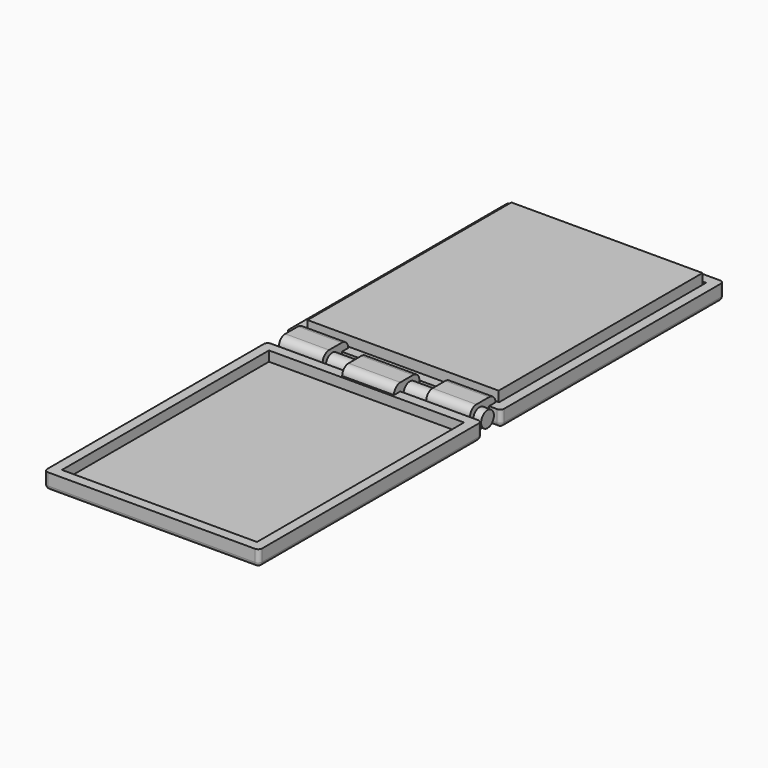
from build123d import *

# Parameters (mm, degrees)
F0_W      = 24
F0_H      = 32
F1_DEPTH  = 2.1
F3_W      = 27.0000016689
F3_H      = 35.0000016689
F3_W_2    = 24
F3_H_2    = 32
F4_DEPTH  = 4
F6_OFFSET = 0.25
F7_R      = 0.5
F5_W      = 35.0000016689
F5_H      = 2
F8_DEPTH  = 27.0000016689
F11_W     = 6.5
F11_H     = 2.9999983311
F11_H_2   = 1
F12_DEPTH = 3
F11_W_2   = 5.5000003338
F11_W_3   = 5.5000004172
F13_R     = 1
F14_DEPTH = 25
F15_R     = 1
F15_2_R   = 1
F15_3_R   = 1


with BuildPart() as f1:
    # F0 (on Top) → F1 (new body)
    with BuildSketch(Plane.XY):
        with Locations((12, 16)):
            Rectangle(F0_W, F0_H)
    extrude(amount=F1_DEPTH)


with BuildPart() as f4:
    # F3 (on offset) → F4 (new body)
    with BuildSketch(Plane.XY.offset(-1)):
        with Locations((12, 16)):
            Rectangle(F3_W, F3_H)
        with Locations((12, 16)):
            Rectangle(F3_W_2, F3_H_2, mode=Mode.SUBTRACT)
        with Locations((12, 16)):
            Rectangle(F3_W_2, F3_H_2)
    extrude(amount=F4_DEPTH)

    # F6: cut F1, made larger all round first
    f6_tool = offset(f1.part, amount=F6_OFFSET, kind=Kind.INTERSECTION, mode=Mode.PRIVATE)
    add(f6_tool, mode=Mode.SUBTRACT)

    # F7
    f7_edges = [f4.edges().sort_by_distance(p)[0] for p in [
        (-1.500001, -1.500001, 1),
        (25.500001, -1.500001, 1),
        (25.500001, 33.500001, 1),
        (-1.500001, 33.500001, 1),
        (-1.500001, 16, 3),
        (12, 33.500001, 3),
        (12, 33.500001, -1),
        (-1.500001, 16, -1),
        (25.500001, 16, 3),
        (25.500001, 16, -1),
        (12, -1.500001, 3),
        (12, -1.500001, -1),
    ]]
    fillet(f7_edges, radius=F7_R)

    # F5 (on face) → F8 (cut, through all)
    with BuildSketch(Plane.YZ.offset(25.5000008345)):
        with Locations((16, 2)):
            Rectangle(F5_W, F5_H)
    extrude(amount=-F8_DEPTH, mode=Mode.SUBTRACT)


with BuildPart() as f10_1:
    # F10: instance of F4
    add(f4.part.mirror(Plane.XZ.offset(3)))


with BuildPart() as f12:
    # F11 (on offset) → F12 (new body)
    with BuildSketch(Plane.XY.offset(-1)):
        with Locations((11.9999995828, -3)):
            Rectangle(F11_W, F11_H)
        with Locations((11.9999995828, -4.9999991655)):
            Rectangle(F11_W, F11_H_2)
    extrude(amount=F12_DEPTH)

    # F15
    f15_edges = [f12.edges().sort_by_distance(p)[0] for p in [
        (12, -5.499999, 2),
        (12, -1.500001, 2),
    ]]
    fillet(f15_edges, radius=F15_R)


with BuildPart() as f12b:
    # F11 (on offset) → F12, piece 2 (new body)
    with BuildSketch(Plane.XY.offset(-1)):
        with Locations((21.2500005841, -3)):
            Rectangle(F11_W_2, F11_H)
        with Locations((21.2500006258, -1.0000008345)):
            Rectangle(F11_W_3, F11_H_2)
    extrude(amount=F12_DEPTH)

    # F15#2
    f15_2_edges = [f12b.edges().sort_by_distance(p)[0] for p in [
        (21.250001, -0.500001, 2),
        (21.25, -4.499999, 2),
    ]]
    fillet(f15_2_edges, radius=F15_2_R)


with BuildPart() as f12c:
    # F11 (on offset) → F12, piece 3 (new body)
    with BuildSketch(Plane.XY.offset(-1)):
        with Locations((2.7499993742, -1.0000008345)):
            Rectangle(F11_W_3, F11_H_2)
        Polygon((5.4999995828, -1.5000008345), (-6.676e-07, -1.5000008345), (0, -4.4999991655), (5.4999995828, -4.4999991655), align=None)
    extrude(amount=F12_DEPTH)

    # F15#3
    f15_3_edges = [f12c.edges().sort_by_distance(p)[0] for p in [
        (2.749999, -0.500001, 2),
        (2.75, -4.499999, 2),
    ]]
    fillet(f15_3_edges, radius=F15_3_R)


with BuildPart() as f14:
    # F13 (on face) → F14 (new body)
    with BuildSketch(Plane(origin=(-9.179e-07, 0, 0), x_dir=(1.669e-07, -1, 0), z_dir=(-1, -1.669e-07, 0))):
        with Locations((3, 0.5)):
            Circle(F13_R)
    extrude(amount=-F14_DEPTH)


solid = Compound([f1.part, f4.part, f10_1.part, f12.part, f12b.part, f12c.part, f14.part])
